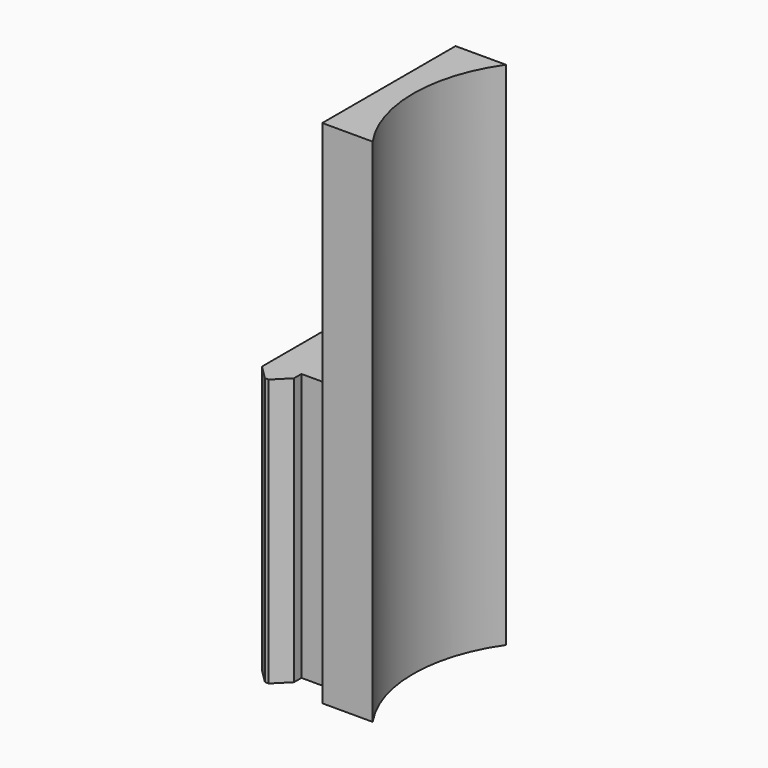
from build123d import *

# Parameters (mm, degrees)
F0_W     = 5.1562
F0_H     = 7.8232
F1_DEPTH = 34.925
F2_DEPTH = 31.75


with BuildPart() as f1:
    # F0 (on Top) → F1 (new body)
    with BuildSketch(Plane.XY):
        with BuildLine():
            Line((2.8402731368, 10.8712), (0, 10.8712))
            Line((0, 10.8712), (0, 7.8232))
            Line((0, 7.8232), (0, 0))
            ThreePointArc((0, 0), (0.7217888499, 5.6180543993), (2.8402731368, 10.8712))
        make_face()
        with Locations((-2.5781, 3.9116)):
            Rectangle(F0_W, F0_H)
        with BuildLine():
            Line((6.5814866299, 10.8712), (2.8402731368, 10.8712))
            ThreePointArc((2.8402731368, 10.8712), (0.7217888499, 5.6180543993), (0, 0))
            ThreePointArc((0, 0), (0.7217888499, -5.6180543993), (2.8402731368, -10.8712))
            Line((2.8402731368, -10.8712), (6.5814866299, -10.8712))
            ThreePointArc((6.5814866299, -10.8712), (3.175, 0), (6.5814866299, 10.8712))
        make_face()
        with BuildLine():
            ThreePointArc((2.8402731368, -10.8712), (0.7217888499, -5.6180543993), (0, 0))
            Line((0, 0), (0, -7.8232))
            Line((0, -7.8232), (0, -10.8712))
            Line((0, -10.8712), (2.8402731368, -10.8712))
        make_face()
        with Locations((-2.5781, -3.9116)):
            Rectangle(F0_W, F0_H)
        Polygon((-5.1562, 0), (-5.1562, 7.8232), (-5.1562, 9.0424), (-5.8674, 9.7536), (-5.8674, 0), align=None)
        Polygon((-5.8674, 9.7536), (-6.985, 10.8712), (-7.239, 10.8712), (-7.239, 9.7536), align=None)
        Polygon((-5.8674, 0), (-5.8674, 9.7536), (-7.239, 9.7536), (-7.239, 0), (-7.1374, 0), align=None)
        Polygon((-5.1562, -7.8232), (-5.1562, 0), (-5.8674, 0), (-5.8674, -9.7536), (-5.1562, -9.0424), align=None)
        Polygon((-7.239, 9.7536), (-7.239, 10.8712), (-7.493, 10.8712), (-8.6106, 9.7536), align=None)
        Polygon((-7.239, 0), (-7.239, 9.7536), (-8.6106, 9.7536), (-8.6106, 0), (-7.3406, 0), align=None)
        Polygon((-5.8674, -9.7536), (-5.8674, 0), (-7.1374, 0), (-7.239, 0), (-7.239, -9.7536), align=None)
        Polygon((-8.6106, 0), (-8.6106, 9.7536), (-9.3218, 9.0424), (-9.3218, 0), align=None)
        Polygon((-7.239, -9.7536), (-7.239, 0), (-7.3406, 0), (-8.6106, 0), (-8.6106, -9.7536), align=None)
        Polygon((-6.985, -10.8712), (-5.8674, -9.7536), (-7.239, -9.7536), (-7.239, -10.8712), align=None)
        Polygon((-8.6106, -9.7536), (-8.6106, 0), (-9.3218, 0), (-9.3218, -9.0424), align=None)
        Polygon((-7.239, -10.8712), (-7.239, -9.7536), (-8.6106, -9.7536), (-7.493, -10.8712), align=None)
    extrude(amount=-F1_DEPTH)

    # F0 (on Top) → F2 (join)
    with BuildSketch(Plane.XY):
        with BuildLine():
            Line((2.8402731368, 10.8712), (0, 10.8712))
            Line((0, 10.8712), (0, 7.8232))
            Line((0, 7.8232), (0, 0))
            ThreePointArc((0, 0), (0.7217888499, 5.6180543993), (2.8402731368, 10.8712))
        make_face()
        with BuildLine():
            ThreePointArc((2.8402731368, -10.8712), (0.7217888499, -5.6180543993), (0, 0))
            Line((0, 0), (0, -7.8232))
            Line((0, -7.8232), (0, -10.8712))
            Line((0, -10.8712), (2.8402731368, -10.8712))
        make_face()
        with BuildLine():
            Line((6.5814866299, 10.8712), (2.8402731368, 10.8712))
            ThreePointArc((2.8402731368, 10.8712), (0.7217888499, 5.6180543993), (0, 0))
            ThreePointArc((0, 0), (0.7217888499, -5.6180543993), (2.8402731368, -10.8712))
            Line((2.8402731368, -10.8712), (6.5814866299, -10.8712))
            ThreePointArc((6.5814866299, -10.8712), (3.175, 0), (6.5814866299, 10.8712))
        make_face()
    extrude(amount=F2_DEPTH)


with BuildPart() as f3_1:
    # F3: copy of F1
    add(f1.part)


solid = Compound([f1.part, f3_1.part])
